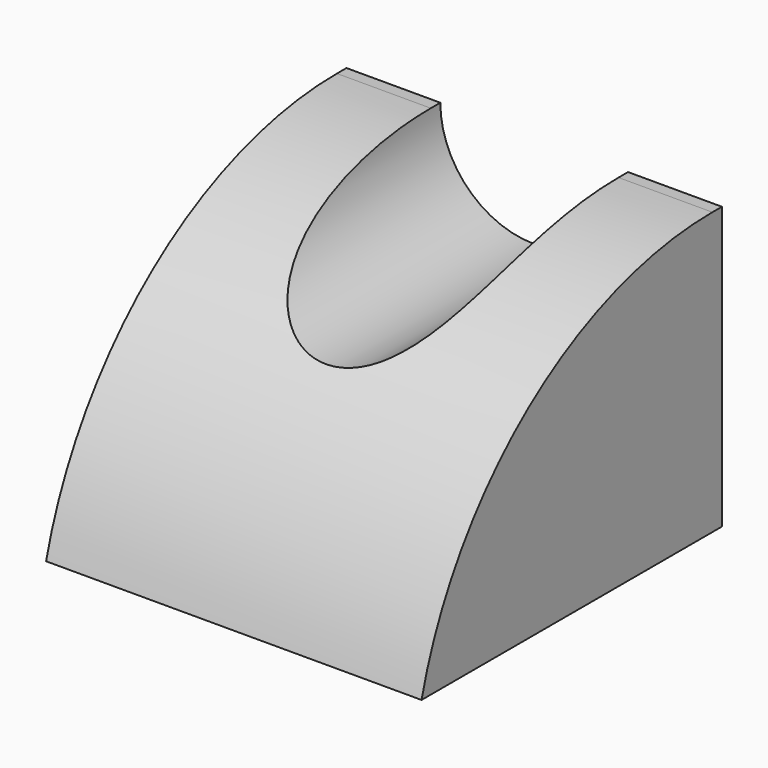
from build123d import *

# Parameters (mm, degrees)
F1_DEPTH    = 50
F2_T1_DEPTH = 509.1229182759
F3_T        = -2


# Not quite as in the source:
# - a fillet or chamfer that OpenCascade refuses, or shapes differently, is made with other operations: its cross-section is extruded or revolved along the edge and cut away or added


with BuildPart() as f1:
    # F0 (on Front) → F1 (new body, symmetric)
    with BuildSketch(Plane.XZ):
        with BuildLine():
            Line((50, -37.5), (50, 37.5))
            Line((50, 37.5), (25, 37.5))
            ThreePointArc((25, 37.5), (0, 12.5), (-25, 37.5))
            Line((-25, 37.5), (-50, 37.5))
            Line((-50, 37.5), (-50, -37.5))
            Line((-50, -37.5), (50, -37.5))
        make_face()
    extrude(amount=F1_DEPTH, both=True)

    # F2: fillet of radius 100 on 1 edges, made by hand

    # F2_s2 → F2_t1 (cut)
    with BuildSketch(Plane.YZ.offset(-217.061459138)):
        with BuildLine():
            ThreePointArc((-50, -37.5), (-14.4126599144, 16.5569415042), (46.8245836552, 37.5))
            Line((46.8245836552, 37.5), (-50, 37.5))
            Line((-50, 37.5), (-50, -37.5))
        make_face()
    extrude(amount=F2_T1_DEPTH, mode=Mode.SUBTRACT)

    # F3
    f3_openings = [f1.faces().sort_by_distance(p)[0] for p in [
        (0, 50, -4.049992),
        (0, 0, -37.5),
    ]]
    offset(amount=F3_T, openings=f3_openings, kind=Kind.INTERSECTION)


solid = f1.part
